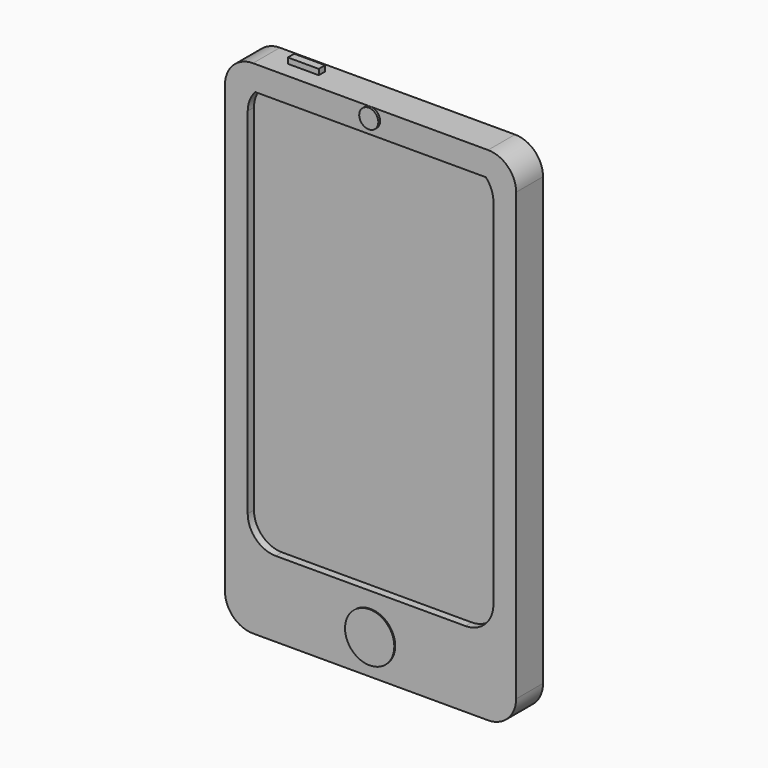
from build123d import *

# Parameters (mm, degrees)
F1_DEPTH   = 7.62
F3_DEPTH   = 1.778
F4_R       = 5.5910358915
F6_DEPTH   = 0.254
F11_W      = 5.8401450515
F11_H      = 0.8899270086
F12_DEPTH  = 0.254
F13_W      = 53.3195276141
F13_H      = 7.62
F13_W_2    = 3.7960950285
F13_H_2    = 0.8621166
F14_DEPTH  = 5.588
F15_W      = 5.4543595761
F15_H      = 1.4679813758
F16_DEPTH  = 2.921
F17_W      = 7.0071518421
F17_H      = 1.8082973547
F18_DEPTH  = 1.27
F19_R      = 2.1642296788
F20_DEPTH  = 0.508
F21_R      = 3.8279673228
F22_DEPTH  = 2.286
F23_R      = 4.5034446875
F23_R_2    = 3.1940667159
F24_DEPTH  = 0.6604
F26_W      = 9.0522272512
F26_H      = 1.7520438414
F27_DEPTH  = 12.192
F1_FACE2_W = 53.3195276141
F1_FACE2_H = 7.62
F28_DEPTH  = 1.27
F29_W      = 17.2284310684
F29_H      = 1.4600362629
F30_DEPTH  = 3.048
F31_W      = 53.3195276141
F31_H      = 7.62
F31_W_2    = 12.5563140027
F31_H_2    = 1.4600367285
F32_DEPTH  = 1.27
F33_W      = 30.4326713085
F33_H      = 2.039485611
F34_DEPTH  = 1.27
F35_DEPTH  = 2.667


# Not quite as in the source:
# - a fillet or chamfer that OpenCascade refuses, or shapes differently, is made with other operations: its cross-section is extruded or revolved along the edge and cut away or added
# - the program builds the solid bodies; features that only make, move or delete a surface that nothing else refers to are left out


with BuildPart() as f1:
    # F0 (on Front) → F1 (new body)
    with BuildSketch(Plane.XZ):
        with BuildLine():
            ThreePointArc((33.0097638071, 50.5758779287), (31.1498918676, 55.0660059893), (26.6597638071, 56.9258779287))
            Line((26.6597638071, 56.9258779287), (-26.6597638071, 56.9258779287))
            ThreePointArc((-26.6597638071, 56.9258779287), (-31.1498918676, 55.0660059893), (-33.0097638071, 50.5758779287))
            Line((-33.0097638071, 50.5758779287), (-33.0097638071, -50.5758779287))
            ThreePointArc((-33.0097638071, -50.5758779287), (-31.1498918676, -55.0660059893), (-26.6597638071, -56.9258779287))
            Line((-26.6597638071, -56.9258779287), (26.6597638071, -56.9258779287))
            ThreePointArc((26.6597638071, -56.9258779287), (31.1498918676, -55.0660059893), (33.0097638071, -50.5758779287))
            Line((33.0097638071, -50.5758779287), (33.0097638071, 50.5758779287))
        make_face()
    extrude(amount=F1_DEPTH)

    # F2 (on face) → F3 (cut)
    with BuildSketch(Plane.XZ.offset(7.62)):
        with BuildLine():
            ThreePointArc((27.8582237661, 46.9814757049), (25.9983518266, 51.4716037654), (21.5082237661, 53.3314757049))
            Line((21.5082237661, 53.3314757049), (-21.5082237661, 53.3314757049))
            ThreePointArc((-21.5082237661, 53.3314757049), (-25.9983518266, 51.4716037654), (-27.8582237661, 46.9814757049))
            Line((-27.8582237661, 46.9814757049), (-27.8582237661, -33.4204429924))
            ThreePointArc((-27.8582237661, -33.4204429924), (-25.9983518266, -37.910571053), (-21.5082237661, -39.7704429924))
            Line((-21.5082237661, -39.7704429924), (21.5082237661, -39.7704429924))
            ThreePointArc((21.5082237661, -39.7704429924), (25.9983518266, -37.910571053), (27.8582237661, -33.4204429924))
            Line((27.8582237661, -33.4204429924), (27.8582237661, 46.9814757049))
        make_face()
    extrude(amount=-F3_DEPTH, mode=Mode.SUBTRACT)

    # F4 (on face) → F6 (join)
    with BuildSketch(Plane.XZ.offset(7.62)):
        with Locations((0, -48.9313825965)):
            Circle(F4_R)
    extrude(amount=F6_DEPTH)

    # F11 (on face) → F12 (join)
    with BuildSketch(Plane.XY.offset(56.9258779287)):
        with Locations((20.8248868585, -3.3650364957)):
            Rectangle(F11_W, F11_H)
    extrude(amount=-F12_DEPTH)

    # F13 (on face) → F14 (join)
    with BuildSketch(Plane.XY.offset(56.9258779287)):
        with Locations((0, -3.81)):
            Rectangle(F13_W, F13_H)
        with Locations((21.5549049899, -4.2410583)):
            Rectangle(F13_W_2, F13_H_2, mode=Mode.SUBTRACT)
    extrude(amount=-F14_DEPTH)

    # F15 (on face) → F16 (join)
    with BuildSketch(Plane.XY.offset(56.9258779287)):
        with Locations((18.7206258997, -3.3238437027)):
            Rectangle(F15_W, F15_H)
    extrude(amount=-F16_DEPTH)

    # F17 (on face) → F18 (join)
    with BuildSketch(Plane.XY.offset(56.9258779287)):
        with Locations((-18.1839093566, -3.046388505)):
            Rectangle(F17_W, F17_H)
    extrude(amount=F18_DEPTH)

    # F19 (on face) → F20 (join)
    with BuildSketch(Plane.XZ.offset(7.62)):
        with Locations((0, 54.7479093075)):
            Circle(F19_R)
    extrude(amount=F20_DEPTH)

    # F21 (on face) → F22 (join)
    with BuildSketch(Plane(origin=(0, 0, 0), x_dir=(-1, 0, 0), z_dir=(0, 1, 0))):
        with Locations((24.0557044744, 50.6977252662)):
            Circle(F21_R)
    extrude(amount=-F22_DEPTH)

    # F26 (on face) → F27 (join)
    with BuildSketch(Plane(origin=(0, 0, -56.9258779287), x_dir=(1, 0, 0), z_dir=(0, 0, -1))):
        with Locations((1.1143940501, 4.3801093707)):
            Rectangle(F26_W, F26_H)
    extrude(amount=-F27_DEPTH)

    # F1_face2 (on face) + F26 (on face) → F28 (join)
    with BuildSketch(Plane(origin=(0, -3.81, -56.9258779287), x_dir=(1, 0, 0), z_dir=(0, 0, -1))):
        Rectangle(F1_FACE2_W, F1_FACE2_H)
    with BuildSketch(Plane(origin=(0, 0, -56.9258779287), x_dir=(1, 0, 0), z_dir=(0, 0, -1))):
        with Locations((1.1143940501, 4.3801093707)):
            Rectangle(F26_W, F26_H)
    extrude(amount=-F28_DEPTH)

    # F29 (on face) → F30 (join)
    with BuildSketch(Plane(origin=(0, 0, -56.9258779287), x_dir=(1, 0, 0), z_dir=(0, 0, -1))):
        with Locations((1.1143931188, 4.52611316)):
            Rectangle(F29_W, F29_H)
    extrude(amount=-F30_DEPTH)

    # F31 (on face) → F32 (join)
    with BuildSketch(Plane(origin=(0, 0, -56.9258779287), x_dir=(1, 0, 0), z_dir=(0, 0, -1))):
        with Locations((0, 3.81)):
            Rectangle(F31_W, F31_H)
        with Locations((2.5744300801, 4.8181207385)):
            Rectangle(F31_W_2, F31_H_2, mode=Mode.SUBTRACT)
    extrude(amount=-F32_DEPTH)

    # F33 (on face) → F34 (join)
    with BuildSketch(Plane(origin=(0, 0, -56.9258779287), x_dir=(1, 0, 0), z_dir=(0, 0, -1))):
        with Locations((0, 4.492924083)):
            Rectangle(F33_W, F33_H)
    extrude(amount=F34_DEPTH)

    # F35 (cut): a face of the model
    f35_faces = [f1.faces().sort_by_distance(p)[0] for p in [
        (0, -4.492924083, -58.1958779287),
    ]]
    extrude(f35_faces, amount=-F35_DEPTH, mode=Mode.SUBTRACT)


with BuildPart() as f24:
    # F23 (on face) → F24 (new body)
    with BuildSketch(Plane(origin=(0, 0, 0), x_dir=(-1, 0, 0), z_dir=(0, 1, 0))):
        with Locations((18.6664909124, 47.739546746)):
            Circle(F23_R)
        with Locations((18.6664909124, 47.739546746)):
            Circle(F23_R_2, mode=Mode.SUBTRACT)
    extrude(amount=F24_DEPTH)

    # F25: fillet of radius 1.27 on 1 edges, made by hand

    # F25_s1 → F25_t2 (revolve, cut)
    with BuildSketch(Plane.XY.offset(47.739546746)):
        with BuildLine():
            ThreePointArc((-23.1699356, 0), (-22.7033800985, 0.4828953089), (-22.0558046202, 0.6604))
            Line((-22.0558046202, 0.6604), (-23.1699356, 0.6604))
            Line((-23.1699356, 0.6604), (-23.1699356, 0))
        make_face()
    revolve(axis=Axis((-18.6664909124, 0.6604, 47.739546746), (0, 1, 0)), mode=Mode.SUBTRACT)


solid = Compound([f1.part, f24.part])
